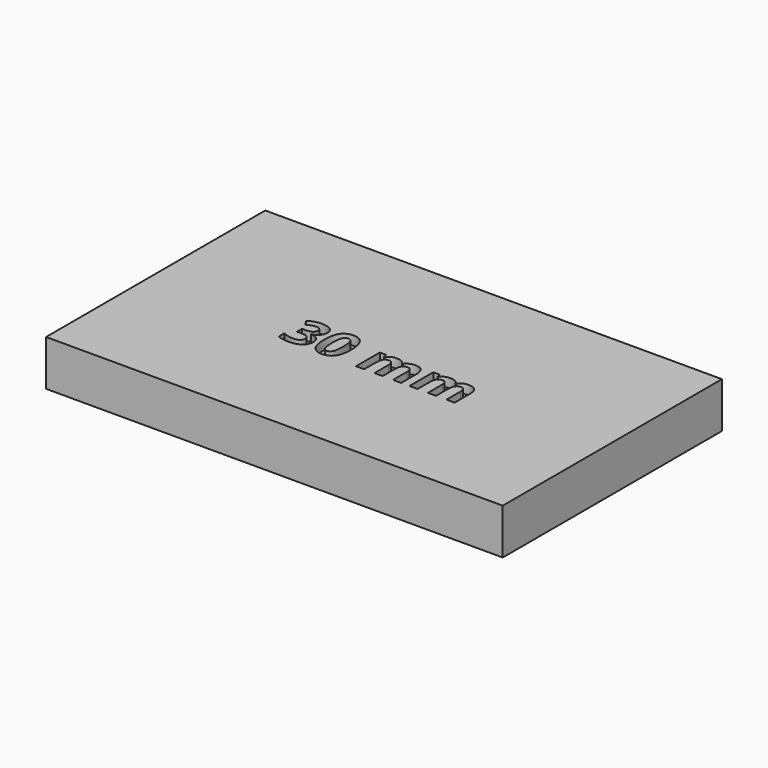
from build123d import *

# Parameters (mm, degrees)
F0_W         = 50
F0_H         = 30
F1_DEPTH     = 5
F2_TEXT_SIZE = 5.9606966564
F3_DEPTH     = 1


# Not quite as in the source:
# - Text() gives the source's letters only with a copy of the font that has no kerning and outlines rounded to 1/6400 em; it was checked with that copy


with BuildPart() as f1:
    # F0 (on Top) → F1 (new body)
    with BuildSketch(Plane.XY):
        with Locations((-25, 15)):
            Rectangle(F0_W, F0_H)
    extrude(amount=F1_DEPTH)

    # F2 (on face) → F3 (cut)
    with BuildSketch(Plane.XY.offset(5)):
        with Locations((-34.7424356574, 12.3251881452)):
            Text('30 mm', F2_TEXT_SIZE, font='Open Sans', font_style=FontStyle.BOLD, text_align=(TextAlign.LEFT, TextAlign.BOTTOM))
    extrude(amount=-F3_DEPTH, mode=Mode.SUBTRACT)


solid = f1.part
